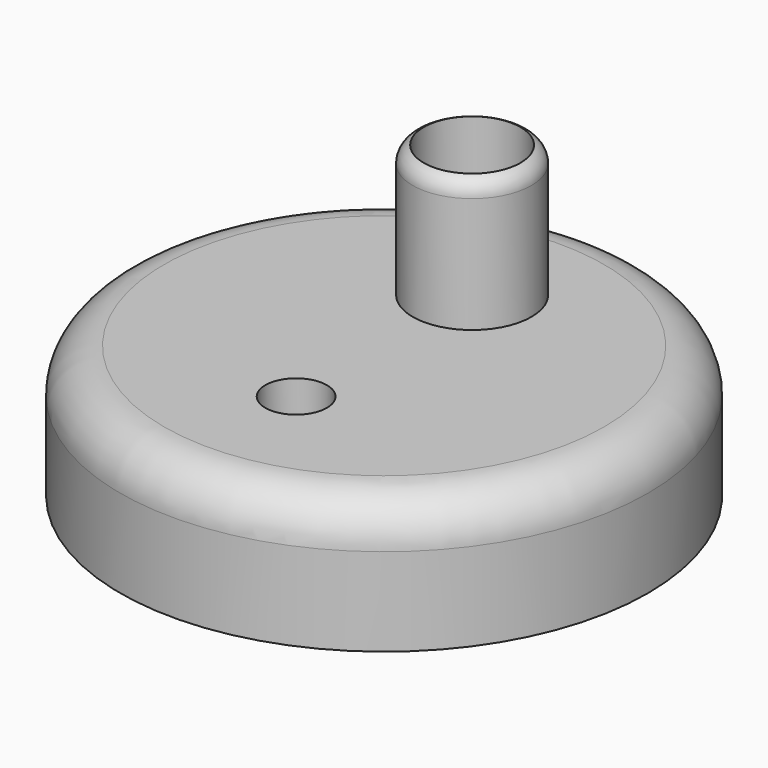
from build123d import *

# Parameters (mm, degrees)
F2_R     = 13.5
F2_R_2   = 11
F3_DEPTH = 30
F5_R     = 7
F6_DEPTH = 10


# Not quite as in the source:
# - a fillet or chamfer that OpenCascade refuses, or shapes differently, is made with other operations: its cross-section is extruded or revolved along the edge and cut away or added


with BuildPart() as f1:
    # F0 (on Front) → F1 (revolve)
    with BuildSketch(Plane.XZ):
        with BuildLine():
            Line((0, 30), (0, 0))
            Line((0, 0), (60, 0))
            Line((60, 0), (60, 20))
            ThreePointArc((60, 20), (57.0710678119, 27.0710678119), (50, 30))
            Line((50, 30), (0, 30))
        make_face()
    revolve(axis=Axis((0, 0, 15), (0, 0, 1)))

    # F2 (on face) → F3 (join)
    with BuildSketch(Plane.XY.offset(30)):
        with Locations((0, 25)):
            Circle(F2_R)
        with Locations((0, 25)):
            Circle(F2_R_2, mode=Mode.SUBTRACT)
    extrude(amount=F3_DEPTH)

    # F4: fillet of radius 4 on 1 edges, made by hand

    # F4_s1 → F4_t2 (revolve, cut)
    with BuildSketch(Plane.XZ.offset(-25)):
        with BuildLine():
            ThreePointArc((13.5, 56.2919007565), (12.8166247904, 58.527968734), (11, 60))
            Line((11, 60), (13.5, 60))
            Line((13.5, 60), (13.5, 56.2919007565))
        make_face()
    revolve(axis=Axis((0, 25, 60), (0, 0, 1)), mode=Mode.SUBTRACT)

    # F5 (on face) → F6 (cut)
    with BuildSketch(Plane.XY.offset(30)):
        with Locations((0, -25)):
            Circle(F5_R)
    extrude(amount=-F6_DEPTH, mode=Mode.SUBTRACT)


solid = f1.part
